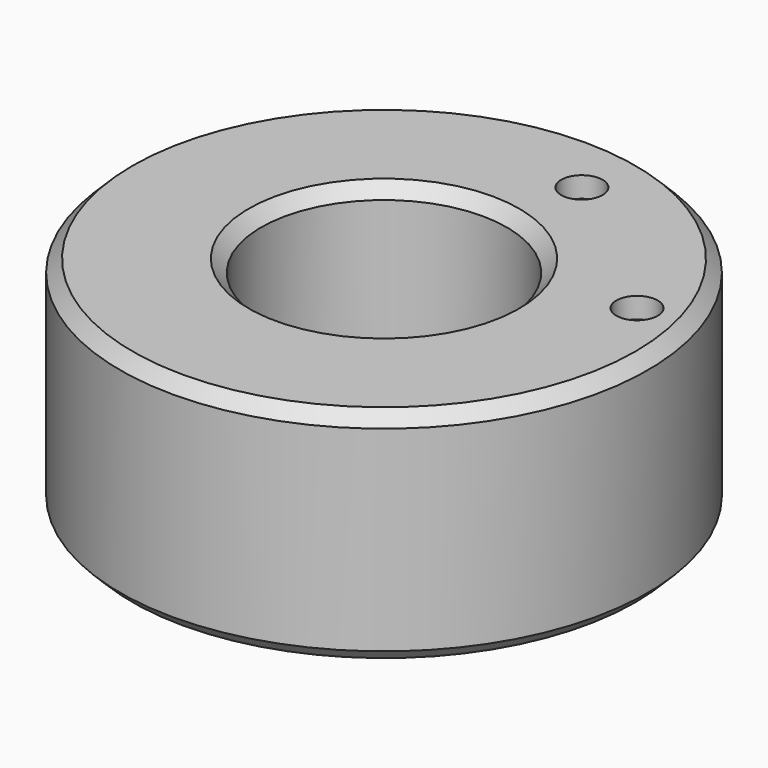
from build123d import *

# Parameters (mm, degrees)
F3_D           = 5
F3_CBORE_D     = 10
F3_CBORE_DEPTH = 5
F4_T6_ANGLE    = 291.5048547237
F4_T14_ANGLE   = 80.1015252238


# Not quite as in the source:
# - a fillet or chamfer that OpenCascade refuses, or shapes differently, is made with other operations: its cross-section is extruded or revolved along the edge and cut away or added


with BuildPart() as f1:
    # F0 (on Right) → F1 (revolve)
    with BuildSketch(Plane.YZ):
        Polygon((63.7261494994, 30.5484924465), (29.6720992774, 30.5484924465), (29.6720992774, -22.7861702442), (41.941575706, -22.7861702442), (41.941575706, -14.2726562917), (51.7070740461, -14.2726562917), (51.7070740461, -22.7861702442), (63.7261494994, -22.7861702442), align=None)
    revolve(axis=Axis((0, 0, 14.0182273462), (0, 0, 1)))

    # F3 (through all)
    with Locations(Plane.XY.offset(30.5484924465)):
        with Locations((10.9902555123, 46.0034860298), (49.8999916017, 14.0128545463)):
            CounterBoreHole(F3_D / 2, F3_CBORE_D / 2, F3_CBORE_DEPTH)

    # F4: chamfer of 3 on 7 edges, made by hand

    # F4_s1 → F4_t2 (revolve, cut)
    with BuildSketch(Plane.YZ):
        Polygon((60.7261494994, 30.5484924465), (63.7261494994, 27.5484924465), (63.7261494994, 30.5484924465), align=None)
    revolve(axis=Axis((0, 0, 30.5484924465), (0, 0, 1)), mode=Mode.SUBTRACT)

    # F4_s3 → F4_t4 (revolve, cut)
    with BuildSketch(Plane.YZ):
        Polygon((63.7261494994, -19.7861702442), (60.7261494994, -22.7861702442), (63.7261494994, -22.7861702442), align=None)
    revolve(axis=Axis((0, 0, -22.7861702442), (0, 0, 1)), mode=Mode.SUBTRACT)

    # F4_s5 → F4_t6 (revolve, cut)
    with BuildSketch(Plane.YZ):
        Polygon((54.7070740461, -22.7861702442), (51.7070740461, -19.7861702442), (51.7070740461, -22.7861702442), align=None)
    revolve(axis=Axis((0, 0, -22.7861702442), (0, 0, 1)), revolution_arc=F4_T6_ANGLE, mode=Mode.SUBTRACT)

    # F4_s7 → F4_t8 (revolve, cut)
    with BuildSketch(Plane.YZ):
        Polygon((38.941575706, -22.7861702442), (41.941575706, -19.7861702442), (41.941575706, -22.7861702442), align=None)
    revolve(axis=Axis((0, 0, -22.7861702442), (0, 0, 1)), mode=Mode.SUBTRACT)

    # F4_s9 → F4_t10 (revolve, cut)
    with BuildSketch(Plane.YZ):
        Polygon((29.6720992774, -19.7861702442), (32.6720992774, -22.7861702442), (29.6720992774, -22.7861702442), align=None)
    revolve(axis=Axis((0, 0, -22.7861702442), (0, 0, 1)), mode=Mode.SUBTRACT)

    # F4_s11 → F4_t12 (revolve, cut)
    with BuildSketch(Plane.YZ):
        Polygon((32.6720992774, 30.5484924465), (29.6720992774, 27.5484924465), (29.6720992774, 30.5484924465), align=None)
    revolve(axis=Axis((0, 0, 30.5484924465), (0, 0, 1)), mode=Mode.SUBTRACT)

    # F4_s13 → F4_t14 (revolve, cut)
    with BuildSketch(Plane(origin=(0, 0, 0), x_dir=(0, 0, 1), z_dir=(0.1719028764, -0.9851139026, 0))):
        Polygon((-22.7861702442, -54.7070740461), (-19.7861702442, -51.7070740461), (-22.7861702442, -51.7070740461), align=None)
    revolve(axis=Axis((0, 0, -22.7861702442), (0, 0, 1)), revolution_arc=F4_T14_ANGLE, mode=Mode.SUBTRACT)


solid = f1.part
